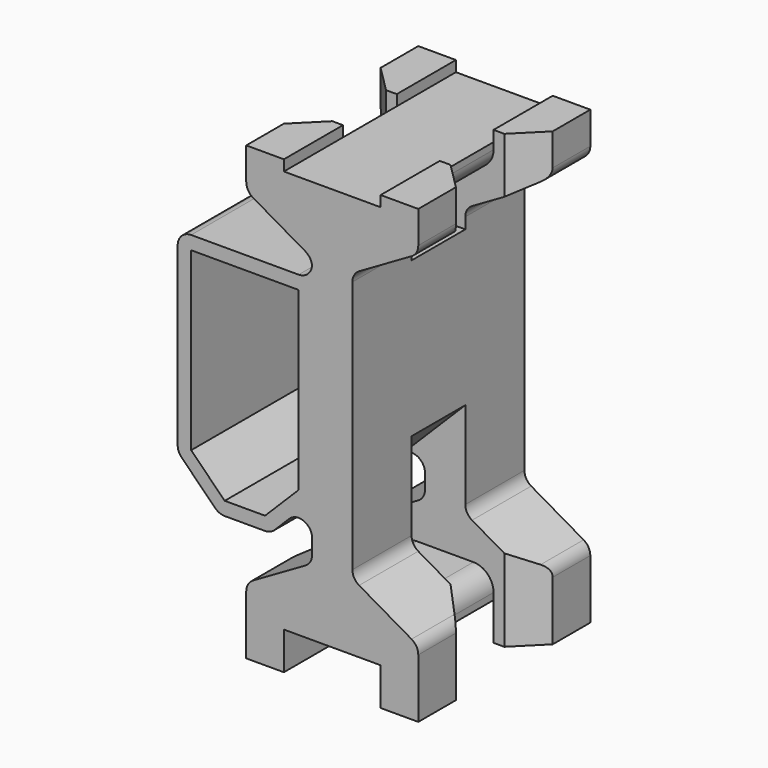
from build123d import *

# Parameters (mm, degrees)
F1_DEPTH      = 16
F2_W          = 2.8
F2_H          = 5
F3_DEPTH      = 33.601
F4_W          = 5
F4_H          = 26
F5_DEPTH      = 10.001
F7_DEPTH      = 16
F8_R          = 1.5
F9_SIZE       = 2
F10_T1_DEPTH  = 5.5
F10_T3_DEPTH  = 5.5
F10_T8_DEPTH  = 11.5355339059
F10_T13_DEPTH = 11.5355339059
F10_T15_DEPTH = 21
F10_T17_DEPTH = 18.0710678119
F10_T19_DEPTH = 6.3867513459
F10_T21_DEPTH = 6.3867513459


# Not quite as in the source:
# - a fillet or chamfer that OpenCascade refuses, or shapes differently, is made with other operations: its cross-section is extruded or revolved along the edge and cut away or added


with BuildPart() as f1:
    # F0 (on Front) → F1 (new body)
    with BuildSketch(Plane.XZ):
        Polygon((-3.6, 30.8), (-6.4, 30.8), (-6.4, 27.829016319), (-1.5, 25), (-1.5, 5), (-6.4, 2.170983681), (-6.4, -2.8), (-3.6, -2.8), (-3.6, 0), (3.6, 0), (3.6, -2.8), (6.4, -2.8), (6.4, 2.170983681), (1.5, 5), (1.5, 25), (6.4, 27.829016319), (6.4, 30.8), (3.6, 30.8), (3.6, 30), (-3.6, 30), align=None)
    extrude(amount=F1_DEPTH)

    # F2 (on face) → F3 (cut, through all)
    with BuildSketch(Plane.XY.offset(30.8)):
        with Locations((-5, -8)):
            Rectangle(F2_W, F2_H)
        with Locations((5, -8)):
            Rectangle(F2_W, F2_H)
    extrude(amount=-F3_DEPTH, mode=Mode.SUBTRACT)

    # F4 (on face) → F5 (cut, through all)
    with BuildSketch(Plane(origin=(-3.6, 0, 0), x_dir=(0, -1, 0), z_dir=(-1, 0, 0))):
        with Locations((8, 15)):
            Rectangle(F4_W, F4_H)
    extrude(amount=-F5_DEPTH, mode=Mode.SUBTRACT)

    # F6 (on face) → F7 (join, through all)
    with BuildSketch(Plane.XZ.offset(16)):
        Polygon((-8.4142135624, 6), (-4.5857864376, 6), (1.5, 12.0857864376), (1.5, 23.6), (-11.5, 23.6), (-11.5, 9.0857864376), align=None)
        Polygon((-10.5, 9.5), (-10.5, 22.6), (-2.5, 22.6), (-2.5, 9.5), (-5, 7), (-8, 7), align=None, mode=Mode.SUBTRACT)
    extrude(amount=-F7_DEPTH)

    # F8
    f8_edges = [f1.edges().sort_by_distance(p)[0] for p in [
        (3.6, -8, 2),
        (3.6, -8, 28),
        (-3.6, -8, 28),
        (-3.6, -8, 2),
    ]]
    fillet(f8_edges, radius=F8_R)

    # F9
    f9_edges = [f1.edges().sort_by_distance(p)[0] for p in [
        (6.4, -10.5, -0.314508),
        (6.4, -5.5, -0.314508),
        (6.4, -10.5, 29.314508),
        (6.4, -5.5, 29.314508),
        (-6.4, -5.5, -0.314508),
        (-6.4, -10.5, -0.314508),
        (-6.4, -5.5, 29.314508),
        (-6.4, -10.5, 29.314508),
    ]]
    chamfer(f9_edges, length=F9_SIZE)

    # F10: fillet of radius 1 on 24 edges, made by hand

    # F10_s2 → F10_t1 (join)
    with BuildSketch(Plane.XZ.offset(10.5)):
        with BuildLine():
            ThreePointArc((-3.2071067812, 7.3786796564), (-2.1173165676, 7.5954524078), (-1.5, 6.6715728753))
            Line((-1.5, 6.6715728753), (-1.5, 9.0857864376))
            Line((-1.5, 9.0857864376), (-3.2071067812, 7.3786796564))
        make_face()
        with BuildLine():
            ThreePointArc((-1.5, 24.6), (-1.7928932188, 23.8928932188), (-2.5, 23.6))
            Line((-2.5, 23.6), (-1.5, 23.6))
            Line((-1.5, 23.6), (-1.5, 24.6))
        make_face()
        with BuildLine():
            ThreePointArc((1.5, 5.5773502692), (1.6339745962, 5.0773502692), (2, 4.7113248654))
            Line((2, 4.7113248654), (1.5, 5))
            Line((1.5, 5), (1.5, 5.5773502692))
        make_face()
        with BuildLine():
            ThreePointArc((1.5, 24.4226497308), (1.6339745962, 24.9226497308), (2, 25.2886751346))
            Line((2, 25.2886751346), (1.5, 25))
            Line((1.5, 25), (1.5, 24.4226497308))
        make_face()
        with BuildLine():
            ThreePointArc((-1.5, 5.5773502692), (-1.6339745962, 5.0773502692), (-2, 4.7113248654))
            Line((-2, 4.7113248654), (-1.5, 5))
            Line((-1.5, 5), (-1.5, 5.5773502692))
        make_face()
        with BuildLine():
            ThreePointArc((-2, 25.2886751346), (-1.6339745962, 24.9226497308), (-1.5, 24.4226497308))
            Line((-1.5, 24.4226497308), (-1.5, 25))
            Line((-1.5, 25), (-2, 25.2886751346))
        make_face()
    extrude(amount=F10_T1_DEPTH)

    # F10_s4 → F10_t3 (join)
    with BuildSketch(Plane.XZ):
        with BuildLine():
            ThreePointArc((-3.2071067812, 7.3786796564), (-2.1173165676, 7.5954524078), (-1.5, 6.6715728753))
            Line((-1.5, 6.6715728753), (-1.5, 9.0857864376))
            Line((-1.5, 9.0857864376), (-3.2071067812, 7.3786796564))
        make_face()
        with BuildLine():
            ThreePointArc((-2.5, 23.6), (-1.7928932188, 23.8928932188), (-1.5, 24.6))
            Line((-1.5, 24.6), (-1.5, 23.6))
            Line((-1.5, 23.6), (-2.5, 23.6))
        make_face()
        with BuildLine():
            ThreePointArc((1.5, 5.5773502692), (1.6339745962, 5.0773502692), (2, 4.7113248654))
            Line((2, 4.7113248654), (1.5, 5))
            Line((1.5, 5), (1.5, 5.5773502692))
        make_face()
        with BuildLine():
            ThreePointArc((1.5, 24.4226497308), (1.6339745962, 24.9226497308), (2, 25.2886751346))
            Line((2, 25.2886751346), (1.5, 25))
            Line((1.5, 25), (1.5, 24.4226497308))
        make_face()
        with BuildLine():
            ThreePointArc((-1.5, 5.5773502692), (-1.6339745962, 5.0773502692), (-2, 4.7113248654))
            Line((-2, 4.7113248654), (-1.5, 5))
            Line((-1.5, 5), (-1.5, 5.5773502692))
        make_face()
        with BuildLine():
            ThreePointArc((-1.5, 24.4226497308), (-1.6339745962, 24.9226497308), (-2, 25.2886751346))
            Line((-2, 25.2886751346), (-1.5, 25))
            Line((-1.5, 25), (-1.5, 24.4226497308))
        make_face()
    extrude(amount=F10_T3_DEPTH)


with BuildPart() as f10_tool6:
    # F10_s7 → F10_t8 (new body)
    with BuildSketch(Plane.XZ.offset(16)):
        with BuildLine():
            ThreePointArc((-3.2071067812, 7.3786796564), (-2.1173165676, 7.5954524078), (-1.5, 6.6715728753))
            Line((-1.5, 6.6715728753), (-1.5, 9.0857864376))
            Line((-1.5, 9.0857864376), (-3.2071067812, 7.3786796564))
        make_face()
    extrude(amount=-F10_T8_DEPTH)

    split(bisect_by=Plane.XZ.offset(5.5), keep=Keep.BOTTOM)


with BuildPart() as f1_1:
    add(f1.part)

    # F10_t5: union F10_tool6
    add(f10_tool6.part)


with BuildPart() as f10_tool11:
    # F10_s12 → F10_t13 (new body)
    with BuildSketch(Plane.XZ.offset(11.5355339059)):
        with BuildLine():
            ThreePointArc((-3.2071067812, 7.3786796564), (-2.1173165676, 7.5954524078), (-1.5, 6.6715728753))
            Line((-1.5, 6.6715728753), (-1.5, 9.0857864376))
            Line((-1.5, 9.0857864376), (-3.2071067812, 7.3786796564))
        make_face()
    extrude(amount=-F10_T13_DEPTH)

    split(bisect_by=Plane.XZ.offset(10.5), keep=Keep.TOP)


with BuildPart() as f1_2:
    add(f1_1.part)

    # F10_t10: union F10_tool11
    add(f10_tool11.part)

    # F10_s16 → F10_t15 (cut)
    with BuildSketch(Plane.XZ.offset(-2.5)):
        with BuildLine():
            ThreePointArc((-11.5, 22.6), (-11.2071067812, 23.3071067812), (-10.5, 23.6))
            Line((-10.5, 23.6), (-11.5, 23.6))
            Line((-11.5, 23.6), (-11.5, 22.6))
        make_face()
    extrude(amount=F10_T15_DEPTH, mode=Mode.SUBTRACT)

    # F10_s18 → F10_t17 (cut)
    with BuildSketch(Plane.XZ.offset(-1.0355339059)):
        with BuildLine():
            ThreePointArc((-11.2071067812, 8.7928932188), (-11.4238795325, 9.1173165676), (-11.5, 9.5))
            Line((-11.5, 9.5), (-11.5, 9.0857864376))
            Line((-11.5, 9.0857864376), (-11.2071067812, 8.7928932188))
        make_face()
        with BuildLine():
            ThreePointArc((-8, 6), (-8.3826834324, 6.0761204675), (-8.7071067812, 6.2928932188))
            Line((-8.7071067812, 6.2928932188), (-8.4142135624, 6))
            Line((-8.4142135624, 6), (-8, 6))
        make_face()
        with BuildLine():
            ThreePointArc((-4.2928932188, 6.2928932188), (-4.6173165676, 6.0761204675), (-5, 6))
            Line((-5, 6), (-4.5857864376, 6))
            Line((-4.5857864376, 6), (-4.2928932188, 6.2928932188))
        make_face()
    extrude(amount=F10_T17_DEPTH, mode=Mode.SUBTRACT)

    # F10_s20 → F10_t19 (cut)
    with BuildSketch(Plane.XZ.offset(11.056624327)):
        with BuildLine():
            ThreePointArc((-6.4, 1.5936334118), (-6.2660254038, 2.0936334118), (-5.9, 2.4596588156))
            Line((-5.9, 2.4596588156), (-6.4, 2.170983681))
            Line((-6.4, 2.170983681), (-6.4, 1.5936334118))
        make_face()
        with BuildLine():
            ThreePointArc((-6.4, 28.4063665882), (-6.2660254038, 27.9063665882), (-5.9, 27.5403411844))
            Line((-5.9, 27.5403411844), (-6.4, 27.829016319))
            Line((-6.4, 27.829016319), (-6.4, 28.4063665882))
        make_face()
        with BuildLine():
            ThreePointArc((6.4, 28.4063665882), (6.2660254038, 27.9063665882), (5.9, 27.5403411844))
            Line((5.9, 27.5403411844), (6.4, 27.829016319))
            Line((6.4, 27.829016319), (6.4, 28.4063665882))
        make_face()
        with BuildLine():
            ThreePointArc((5.9, 2.4596588156), (6.2660254038, 2.0936334118), (6.4, 1.5936334118))
            Line((6.4, 1.5936334118), (6.4, 2.170983681))
            Line((6.4, 2.170983681), (5.9, 2.4596588156))
        make_face()
    extrude(amount=F10_T19_DEPTH, mode=Mode.SUBTRACT)

    # F10_s22 → F10_t21 (cut)
    with BuildSketch(Plane.XZ.offset(-1.443375673)):
        with BuildLine():
            ThreePointArc((-6.4, 1.5936334118), (-6.2660254038, 2.0936334118), (-5.9, 2.4596588156))
            Line((-5.9, 2.4596588156), (-6.4, 2.170983681))
            Line((-6.4, 2.170983681), (-6.4, 1.5936334118))
        make_face()
        with BuildLine():
            ThreePointArc((-5.9, 27.5403411844), (-6.2660254038, 27.9063665882), (-6.4, 28.4063665882))
            Line((-6.4, 28.4063665882), (-6.4, 27.829016319))
            Line((-6.4, 27.829016319), (-5.9, 27.5403411844))
        make_face()
        with BuildLine():
            ThreePointArc((6.4, 28.4063665882), (6.2660254038, 27.9063665882), (5.9, 27.5403411844))
            Line((5.9, 27.5403411844), (6.4, 27.829016319))
            Line((6.4, 27.829016319), (6.4, 28.4063665882))
        make_face()
        with BuildLine():
            ThreePointArc((5.9, 2.4596588156), (6.2660254038, 2.0936334118), (6.4, 1.5936334118))
            Line((6.4, 1.5936334118), (6.4, 2.170983681))
            Line((6.4, 2.170983681), (5.9, 2.4596588156))
        make_face()
    extrude(amount=F10_T21_DEPTH, mode=Mode.SUBTRACT)


solid = f1_2.part
